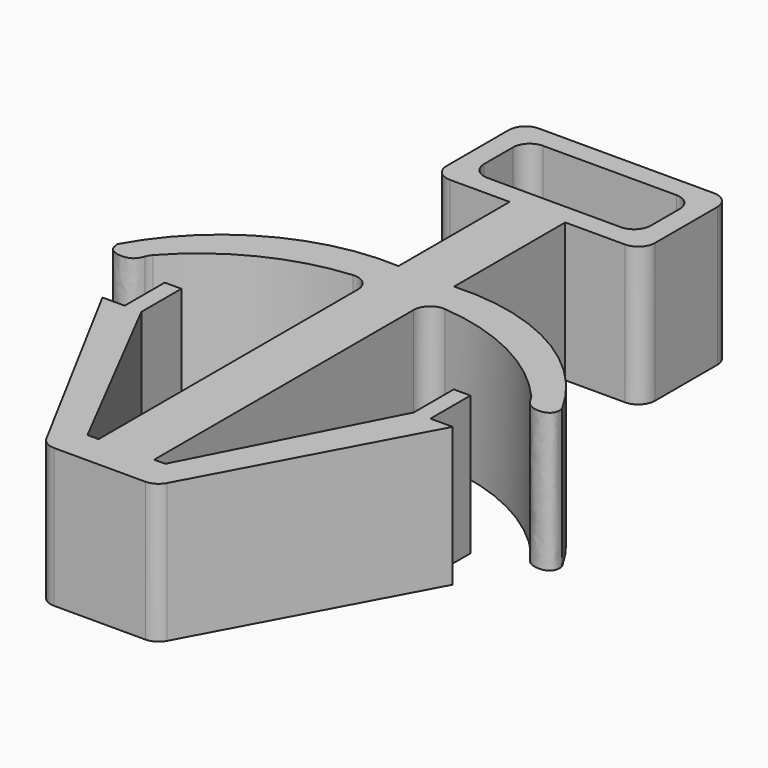
from build123d import *

# Parameters (mm, degrees)
F1_DEPTH = 6.35
F2_R     = 0.762
F4_DEPTH = 6.3510001


with BuildPart() as f1:
    # F0 (on Top) → F1 (new body)
    with BuildSketch(Plane.XY):
        with BuildLine():
            Line((4.7625, 16.3680184094), (-4.7625, 16.3680184094))
            Line((-4.7625, 16.3680184094), (-4.7625, 11.2880184094))
            Line((-4.7625, 11.2880184094), (-1.27, 11.2880184094))
            Line((-1.27, 11.2880184094), (-1.27, 4.9380184094))
            ThreePointArc((-1.27, 4.9380184094), (-6.4291435291, 3.7546941592), (-10.16, 0))
            add(Edge.make_bspline(
                [(-8.7527767482, 0), (-8.8089559621, -0.2418498758), (-9.0471031461, -0.7278683078), (-10.0843877691, -0.5834050266), (-10.1370594903, -0.1969189085), (-10.16, 0)],
                knots=[0, 0, 0, 0, 0.3394019143, 0.707080255, 1, 1, 1, 1], degree=3))
            ThreePointArc((-8.7527767482, 0), (-5.3825469605, 2.5206872974), (-1.27, 3.4147067439))
            Line((-1.27, 3.4147067439), (-1.27, -12.192))
            Line((-1.27, -12.192), (-1.778, -12.192))
            Line((-1.778, -12.192), (-6.223, -3.556))
            Line((-6.223, -3.556), (-6.223, -1.27))
            Line((-6.223, -1.27), (-6.985, -1.27))
            Line((-6.985, -1.27), (-6.985, -3.556))
            Line((-6.985, -3.556), (-8.001, -3.556))
            Line((-8.001, -3.556), (-2.54, -13.716))
            Line((-2.54, -13.716), (2.54, -13.716))
            Line((2.54, -13.716), (8.001, -3.556))
            Line((8.001, -3.556), (6.985, -3.556))
            Line((6.985, -3.556), (6.985, -1.27))
            Line((6.985, -1.27), (6.223, -1.27))
            Line((6.223, -1.27), (6.223, -3.556))
            Line((6.223, -3.556), (1.778, -12.192))
            Line((1.778, -12.192), (1.27, -12.192))
            Line((1.27, -12.192), (1.27, 3.4147067439))
            ThreePointArc((1.27, 3.4147067439), (5.3825469605, 2.5206872974), (8.7527767482, 0))
            add(Edge.make_bspline(
                [(8.7527767482, 0), (8.8795025593, -0.2082938871), (9.0832410123, -0.668988318), (10.0510359017, -0.7151657897), (10.232657896, -0.2924908845), (10.16, 0)],
                knots=[0, 0, 0, 0, 0.3352638068, 0.68469439, 1, 1, 1, 1], degree=3))
            ThreePointArc((10.16, 0), (6.4291435291, 3.7546941592), (1.27, 4.9380184094))
            Line((1.27, 4.9380184094), (1.27, 11.2880184094))
            Line((1.27, 11.2880184094), (4.7625, 11.2880184094))
            Line((4.7625, 11.2880184094), (4.7625, 16.3680184094))
        make_face()
    extrude(amount=F1_DEPTH)

    # F2
    f2_edges = [f1.edges().sort_by_distance(p)[0] for p in [
        (-2.54, -13.716, 3.175),
        (2.54, -13.716, 3.175),
        (-4.7625, 16.368018, 3.175),
        (-4.7625, 11.288018, 3.175),
        (4.7625, 16.368018, 3.175),
        (4.7625, 11.288018, 3.175),
        (1.27, 3.414707, 3.175),
        (8.752777, 0, 3.175),
        (-8.752777, 0, 3.175),
        (-1.27, 3.414707, 3.175),
    ]]
    fillet(f2_edges, radius=F2_R)

    # F3 (on face) → F4 (cut, through all)
    with BuildSketch(Plane.XY.offset(6.35)):
        with BuildLine():
            Line((-3.048, 12.2405184094), (3.048, 12.2405184094))
            ThreePointArc((3.048, 12.2405184094), (3.5868153673, 12.4637030421), (3.81, 13.0025184094))
            Line((3.81, 13.0025184094), (3.81, 14.6535184094))
            ThreePointArc((3.81, 14.6535184094), (3.5868153673, 15.1923337767), (3.048, 15.4155184094))
            Line((3.048, 15.4155184094), (-3.048, 15.4155184094))
            ThreePointArc((-3.048, 15.4155184094), (-3.5868153673, 15.1923337767), (-3.81, 14.6535184094))
            Line((-3.81, 14.6535184094), (-3.81, 13.0025184094))
            ThreePointArc((-3.81, 13.0025184094), (-3.5868153673, 12.4637030421), (-3.048, 12.2405184094))
        make_face()
    extrude(amount=-F4_DEPTH, mode=Mode.SUBTRACT)


solid = f1.part
